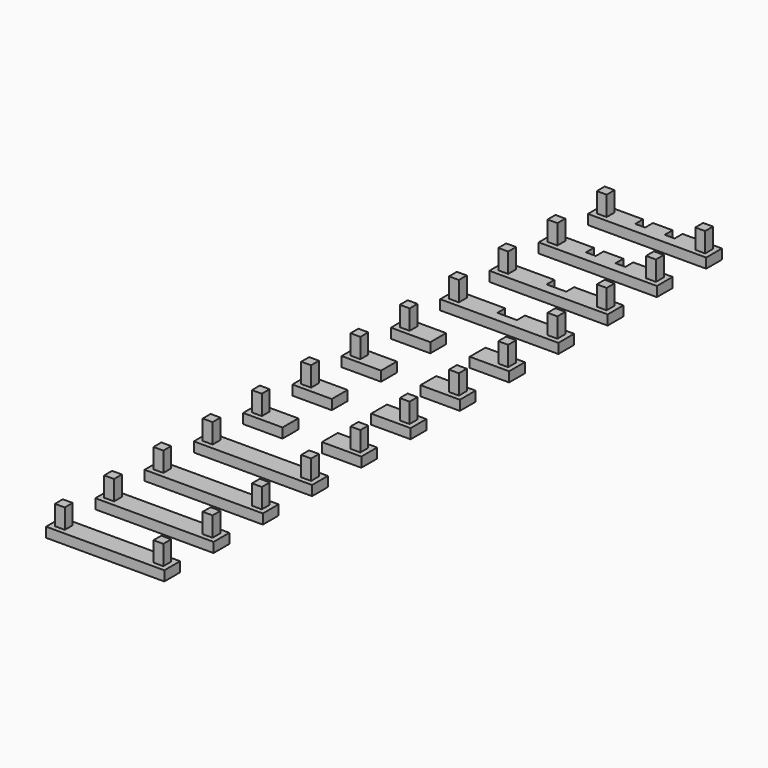
from build123d import *

# Parameters (mm, degrees)
F1_W     = 48
F1_H     = 8
F2_DEPTH = 4
F1_W_2   = 16
F3_W     = 4
F3_H     = 4
F4_DEPTH = 4.001
F5_DEPTH = 8


# Not quite as in the source:
# - a feature names something its author has since deleted; it is built from what else it names


with BuildPart() as f2:
    # F1 (on Top) → F2 (new body)
    with BuildSketch(Plane.XY):
        Rectangle(F1_W, F1_H)
    extrude(amount=F2_DEPTH)


with BuildPart() as f2b:
    # F1 (on Top) → F2, piece 2 (new body)
    with BuildSketch(Plane.XY):
        with Locations((0, 25)):
            Rectangle(F1_W, F1_H)
    extrude(amount=F2_DEPTH)


with BuildPart() as f2c:
    # F1 (on Top) → F2, piece 3 (new body)
    with BuildSketch(Plane.XY):
        with Locations((0, 50)):
            Rectangle(F1_W, F1_H)
    extrude(amount=F2_DEPTH)


with BuildPart() as f2d:
    # F1 (on Top) → F2, piece 4 (new body)
    with BuildSketch(Plane.XY):
        with Locations((0, 75)):
            Rectangle(F1_W, F1_H)
    extrude(amount=F2_DEPTH)


with BuildPart() as f2e:
    # F1 (on Top) → F2, piece 5 (new body)
    with BuildSketch(Plane.XY):
        with Locations((-16, 100)):
            Rectangle(F1_W_2, F1_H)
    extrude(amount=F2_DEPTH)


with BuildPart() as f2f:
    # F1 (on Top) → F2, piece 6 (new body)
    with BuildSketch(Plane.XY):
        with Locations((-16, 125)):
            Rectangle(F1_W_2, F1_H)
    extrude(amount=F2_DEPTH)


with BuildPart() as f2g:
    # F1 (on Top) → F2, piece 7 (new body)
    with BuildSketch(Plane.XY):
        with Locations((-16, 150)):
            Rectangle(F1_W_2, F1_H)
    extrude(amount=F2_DEPTH)


with BuildPart() as f2h:
    # F1 (on Top) → F2, piece 8 (new body)
    with BuildSketch(Plane.XY):
        with Locations((-16, 175)):
            Rectangle(F1_W_2, F1_H)
    extrude(amount=F2_DEPTH)


with BuildPart() as f2i:
    # F1 (on Top) → F2, piece 9 (new body)
    with BuildSketch(Plane.XY):
        with Locations((16, 175)):
            Rectangle(F1_W_2, F1_H)
    extrude(amount=F2_DEPTH)


with BuildPart() as f2j:
    # F1 (on Top) → F2, piece 10 (new body)
    with BuildSketch(Plane.XY):
        with Locations((16, 150)):
            Rectangle(F1_W_2, F1_H)
    extrude(amount=F2_DEPTH)


with BuildPart() as f2k:
    # F1 (on Top) → F2, piece 11 (new body)
    with BuildSketch(Plane.XY):
        with Locations((16, 125)):
            Rectangle(F1_W_2, F1_H)
    extrude(amount=F2_DEPTH)


with BuildPart() as f2l:
    # F1 (on Top) → F2, piece 12 (new body)
    with BuildSketch(Plane.XY):
        with Locations((16, 100)):
            Rectangle(F1_W_2, F1_H)
    extrude(amount=F2_DEPTH)


with BuildPart() as f2m:
    # F1 (on Top) → F2, piece 13 (new body)
    with BuildSketch(Plane.XY):
        Polygon((-24, 204), (-24, 196), (24, 196), (24, 204), (4, 204), (4, 200), (-4, 200), (-4, 204), align=None)
    extrude(amount=F2_DEPTH)


with BuildPart() as f2n:
    # F1 (on Top) → F2, piece 14 (new body)
    with BuildSketch(Plane.XY):
        Polygon((-24, 229), (-24, 221), (24, 221), (24, 229), (4, 229), (4, 225), (-4, 225), (-4, 229), align=None)
    extrude(amount=F2_DEPTH)


with BuildPart() as f2o:
    # F1 (on Top) → F2, piece 15 (new body)
    with BuildSketch(Plane.XY):
        Polygon((-24, 254), (-24, 246), (24, 246), (24, 254), (8, 254), (8, 250), (4, 250), (4, 254), (-4, 254), (-4, 250), (-8, 250), (-8, 254), align=None)
    extrude(amount=F2_DEPTH)


with BuildPart() as f2p:
    # F1 (on Top) → F2, piece 16 (new body)
    with BuildSketch(Plane.XY):
        Polygon((-24, 279), (-24, 271), (24, 271), (24, 279), (8, 279), (8, 275), (4, 275), (4, 279), (-4, 279), (-4, 275), (-8, 275), (-8, 279), align=None)
    extrude(amount=F2_DEPTH)


with BuildPart() as f4_tool:
    # F3 (on face) → F4 (new body, through all)
    with BuildSketch(Plane.XY.offset(4)):
        with Locations((20, 275)):
            Rectangle(F3_W, F3_H)
        with Locations((-20, 275)):
            Rectangle(F3_W, F3_H)
        with Locations((-20, 250)):
            Rectangle(F3_W, F3_H)
        with Locations((20, 250)):
            Rectangle(F3_W, F3_H)
        with Locations((-20, 225)):
            Rectangle(F3_W, F3_H)
        with Locations((20, 225)):
            Rectangle(F3_W, F3_H)
        with Locations((-20, 200)):
            Rectangle(F3_W, F3_H)
        with Locations((20, 200)):
            Rectangle(F3_W, F3_H)
        with Locations((-20, 175)):
            Rectangle(F3_W, F3_H)
        with Locations((20, 175)):
            Rectangle(F3_W, F3_H)
        with Locations((-20, 150)):
            Rectangle(F3_W, F3_H)
        with Locations((20, 150)):
            Rectangle(F3_W, F3_H)
        with Locations((-20, 125)):
            Rectangle(F3_W, F3_H)
        with Locations((20, 125)):
            Rectangle(F3_W, F3_H)
        with Locations((-20, 100)):
            Rectangle(F3_W, F3_H)
        with Locations((20, 100)):
            Rectangle(F3_W, F3_H)
        with Locations((-20, 75)):
            Rectangle(F3_W, F3_H)
        with Locations((20, 75)):
            Rectangle(F3_W, F3_H)
        with Locations((20, 50)):
            Rectangle(F3_W, F3_H)
        with Locations((-20, 50)):
            Rectangle(F3_W, F3_H)
        with Locations((-20, 25)):
            Rectangle(F3_W, F3_H)
        with Locations((20, 25)):
            Rectangle(F3_W, F3_H)
        with Locations((-20, 0)):
            Rectangle(F3_W, F3_H)
        with Locations((20, 0)):
            Rectangle(F3_W, F3_H)
    extrude(amount=-F4_DEPTH)


with BuildPart() as f2_1:
    add(f2.part)

    # F4: cut by f4_tool
    add(f4_tool.part, mode=Mode.SUBTRACT)


with BuildPart() as f2b_1:
    add(f2b.part)

    # F4: cut by f4_tool
    add(f4_tool.part, mode=Mode.SUBTRACT)


with BuildPart() as f2c_1:
    add(f2c.part)

    # F4: cut by f4_tool
    add(f4_tool.part, mode=Mode.SUBTRACT)


with BuildPart() as f2d_1:
    add(f2d.part)

    # F4: cut by f4_tool
    add(f4_tool.part, mode=Mode.SUBTRACT)


with BuildPart() as f2e_1:
    add(f2e.part)

    # F4: cut by f4_tool
    add(f4_tool.part, mode=Mode.SUBTRACT)


with BuildPart() as f2f_1:
    add(f2f.part)

    # F4: cut by f4_tool
    add(f4_tool.part, mode=Mode.SUBTRACT)


with BuildPart() as f2g_1:
    add(f2g.part)

    # F4: cut by f4_tool
    add(f4_tool.part, mode=Mode.SUBTRACT)


with BuildPart() as f2h_1:
    add(f2h.part)

    # F4: cut by f4_tool
    add(f4_tool.part, mode=Mode.SUBTRACT)


with BuildPart() as f2i_1:
    add(f2i.part)

    # F4: cut by f4_tool
    add(f4_tool.part, mode=Mode.SUBTRACT)


with BuildPart() as f2j_1:
    add(f2j.part)

    # F4: cut by f4_tool
    add(f4_tool.part, mode=Mode.SUBTRACT)


with BuildPart() as f2k_1:
    add(f2k.part)

    # F4: cut by f4_tool
    add(f4_tool.part, mode=Mode.SUBTRACT)


with BuildPart() as f2l_1:
    add(f2l.part)

    # F4: cut by f4_tool
    add(f4_tool.part, mode=Mode.SUBTRACT)


with BuildPart() as f2m_1:
    add(f2m.part)

    # F4: cut by f4_tool
    add(f4_tool.part, mode=Mode.SUBTRACT)


with BuildPart() as f2n_1:
    add(f2n.part)

    # F4: cut by f4_tool
    add(f4_tool.part, mode=Mode.SUBTRACT)


with BuildPart() as f2o_1:
    add(f2o.part)

    # F4: cut by f4_tool
    add(f4_tool.part, mode=Mode.SUBTRACT)


with BuildPart() as f2p_1:
    add(f2p.part)

    # F4: cut by f4_tool
    add(f4_tool.part, mode=Mode.SUBTRACT)


with BuildPart() as f5:
    # F3 (on face) → F5 (new body)
    with BuildSketch(Plane.XY.offset(4)):
        with Locations((-20, 0)):
            Rectangle(F3_W, F3_H)
    extrude(amount=F5_DEPTH)


with BuildPart() as f5b:
    # F3 (on face) → F5, piece 2 (new body)
    with BuildSketch(Plane.XY.offset(4)):
        with Locations((20, 0)):
            Rectangle(F3_W, F3_H)
    extrude(amount=F5_DEPTH)


with BuildPart() as f5c:
    # F3 (on face) → F5, piece 3 (new body)
    with BuildSketch(Plane.XY.offset(4)):
        with Locations((20, 25)):
            Rectangle(F3_W, F3_H)
    extrude(amount=F5_DEPTH)


with BuildPart() as f5d:
    # F3 (on face) → F5, piece 4 (new body)
    with BuildSketch(Plane.XY.offset(4)):
        with Locations((-20, 25)):
            Rectangle(F3_W, F3_H)
    extrude(amount=F5_DEPTH)


with BuildPart() as f5e:
    # F3 (on face) → F5, piece 5 (new body)
    with BuildSketch(Plane.XY.offset(4)):
        with Locations((-20, 50)):
            Rectangle(F3_W, F3_H)
    extrude(amount=F5_DEPTH)


with BuildPart() as f5f:
    # F3 (on face) → F5, piece 6 (new body)
    with BuildSketch(Plane.XY.offset(4)):
        with Locations((-20, 75)):
            Rectangle(F3_W, F3_H)
    extrude(amount=F5_DEPTH)


with BuildPart() as f5g:
    # F3 (on face) → F5, piece 7 (new body)
    with BuildSketch(Plane.XY.offset(4)):
        with Locations((20, 75)):
            Rectangle(F3_W, F3_H)
    extrude(amount=F5_DEPTH)


with BuildPart() as f5h:
    # F3 (on face) → F5, piece 8 (new body)
    with BuildSketch(Plane.XY.offset(4)):
        with Locations((20, 50)):
            Rectangle(F3_W, F3_H)
    extrude(amount=F5_DEPTH)


with BuildPart() as f5i:
    # F3 (on face) → F5, piece 9 (new body)
    with BuildSketch(Plane.XY.offset(4)):
        with Locations((20, 100)):
            Rectangle(F3_W, F3_H)
    extrude(amount=F5_DEPTH)


with BuildPart() as f5j:
    # F3 (on face) → F5, piece 10 (new body)
    with BuildSketch(Plane.XY.offset(4)):
        with Locations((-20, 100)):
            Rectangle(F3_W, F3_H)
    extrude(amount=F5_DEPTH)


with BuildPart() as f5k:
    # F3 (on face) → F5, piece 11 (new body)
    with BuildSketch(Plane.XY.offset(4)):
        with Locations((-20, 125)):
            Rectangle(F3_W, F3_H)
    extrude(amount=F5_DEPTH)


with BuildPart() as f5l:
    # F3 (on face) → F5, piece 12 (new body)
    with BuildSketch(Plane.XY.offset(4)):
        with Locations((20, 125)):
            Rectangle(F3_W, F3_H)
    extrude(amount=F5_DEPTH)


with BuildPart() as f5m:
    # F3 (on face) → F5, piece 13 (new body)
    with BuildSketch(Plane.XY.offset(4)):
        with Locations((20, 150)):
            Rectangle(F3_W, F3_H)
    extrude(amount=F5_DEPTH)


with BuildPart() as f5n:
    # F3 (on face) → F5, piece 14 (new body)
    with BuildSketch(Plane.XY.offset(4)):
        with Locations((-20, 150)):
            Rectangle(F3_W, F3_H)
    extrude(amount=F5_DEPTH)


with BuildPart() as f5o:
    # F3 (on face) → F5, piece 15 (new body)
    with BuildSketch(Plane.XY.offset(4)):
        with Locations((-20, 175)):
            Rectangle(F3_W, F3_H)
    extrude(amount=F5_DEPTH)


with BuildPart() as f5p:
    # F3 (on face) → F5, piece 16 (new body)
    with BuildSketch(Plane.XY.offset(4)):
        with Locations((20, 175)):
            Rectangle(F3_W, F3_H)
    extrude(amount=F5_DEPTH)


with BuildPart() as f5q:
    # F3 (on face) → F5, piece 17 (new body)
    with BuildSketch(Plane.XY.offset(4)):
        with Locations((-20, 200)):
            Rectangle(F3_W, F3_H)
    extrude(amount=F5_DEPTH)


with BuildPart() as f5r:
    # F3 (on face) → F5, piece 18 (new body)
    with BuildSketch(Plane.XY.offset(4)):
        with Locations((20, 200)):
            Rectangle(F3_W, F3_H)
    extrude(amount=F5_DEPTH)


with BuildPart() as f5s:
    # F3 (on face) → F5, piece 19 (new body)
    with BuildSketch(Plane.XY.offset(4)):
        with Locations((20, 225)):
            Rectangle(F3_W, F3_H)
    extrude(amount=F5_DEPTH)


with BuildPart() as f5t:
    # F3 (on face) → F5, piece 20 (new body)
    with BuildSketch(Plane.XY.offset(4)):
        with Locations((-20, 225)):
            Rectangle(F3_W, F3_H)
    extrude(amount=F5_DEPTH)


with BuildPart() as f5u:
    # F3 (on face) → F5, piece 21 (new body)
    with BuildSketch(Plane.XY.offset(4)):
        with Locations((-20, 250)):
            Rectangle(F3_W, F3_H)
    extrude(amount=F5_DEPTH)


with BuildPart() as f5v:
    # F3 (on face) → F5, piece 22 (new body)
    with BuildSketch(Plane.XY.offset(4)):
        with Locations((20, 250)):
            Rectangle(F3_W, F3_H)
    extrude(amount=F5_DEPTH)


with BuildPart() as f5w:
    # F3 (on face) → F5, piece 23 (new body)
    with BuildSketch(Plane.XY.offset(4)):
        with Locations((20, 275)):
            Rectangle(F3_W, F3_H)
    extrude(amount=F5_DEPTH)


with BuildPart() as f5x:
    # F3 (on face) → F5, piece 24 (new body)
    with BuildSketch(Plane.XY.offset(4)):
        with Locations((-20, 275)):
            Rectangle(F3_W, F3_H)
    extrude(amount=F5_DEPTH)


solid = Compound([f2_1.part, f2b_1.part, f2c_1.part, f2d_1.part, f2e_1.part, f2f_1.part, f2g_1.part, f2h_1.part, f2i_1.part, f2j_1.part, f2k_1.part, f2l_1.part, f2m_1.part, f2n_1.part, f2o_1.part, f2p_1.part, f5.part, f5b.part, f5c.part, f5d.part, f5e.part, f5f.part, f5g.part, f5h.part, f5i.part, f5j.part, f5k.part, f5l.part, f5m.part, f5n.part, f5o.part, f5p.part, f5q.part, f5r.part, f5s.part, f5t.part, f5u.part, f5v.part, f5w.part, f5x.part])
